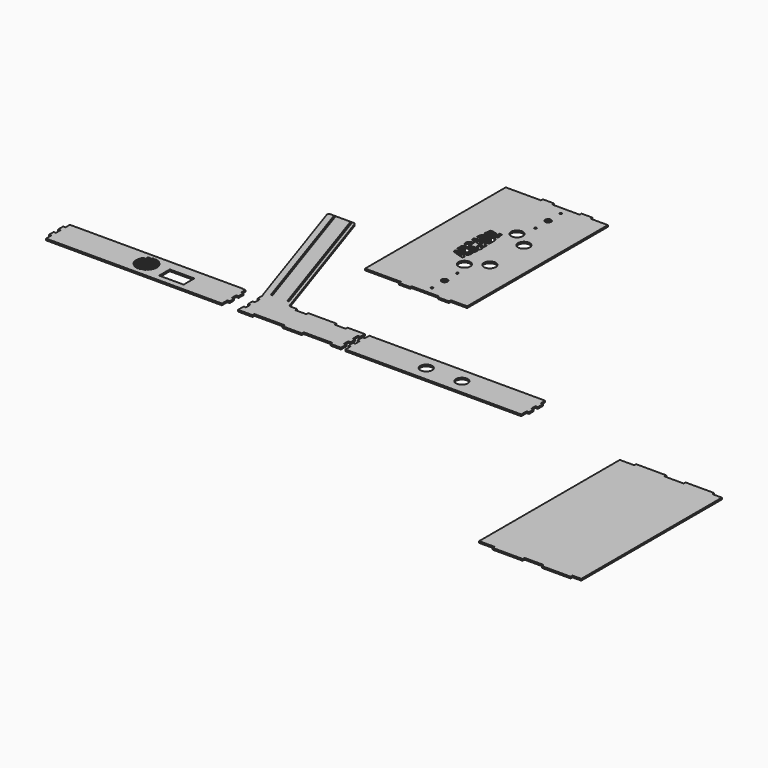
from build123d import *

# Parameters (mm, degrees)
F1_DEPTH = 4.45
F0_R     = 3
F0_R_2   = 8.087272744
F0_R_3   = 16.129
F0_W     = 66.7005181313
F0_H     = 36.3053381443


# Not quite as in the source:
# - ends of sketch curves that miss each other by under 0.0002 mm in the source are joined
# - a feature names something its author has since deleted; it is built from what else it names


with BuildPart() as f1:
    # F0 (on Top) → F1 (new body)
    with BuildSketch(Plane.XY):
        with BuildLine():
            Line((-13.1345508408, -164.6919741164), (-133.2231766972, 195.5739079059))
            ThreePointArc((-133.2231766972, 195.5739079059), (-135.0430417624, 198.0489800139), (-137.9665931933, 198.9927690934))
            Line((-137.9665931933, 198.9927690934), (-188.0199429035, 198.9927690934))
            Line((-188.0199429035, 198.9927690934), (-201.6566259516, 198.9927690934))
            ThreePointArc((-201.6566259516, 198.9927690934), (-205.7128368721, 196.9163205243), (-206.4000424478, 192.4116302809))
            Line((-206.4000424478, 192.4116302809), (-83.9924133672, -174.8112615001))
            Line((-83.9924133672, -174.8112615001), (-80.8544035681, -184.2252910137))
            Line((-80.8544035681, -184.2252910137), (-80.3456279762, -184.2252910137))
            Line((-80.3456279762, -184.2252910137), (-80.3456279762, -185.1425599537))
            Line((-80.3456279762, -185.1425599537), (-80.3456279762, -185.7516178083))
            Line((-80.3456279762, -185.7516178083), (-80.3456279762, -200.4338326941))
            Line((-80.3456279762, -200.4338326941), (-74.0156279762, -200.4338326941))
            Line((-74.0156279762, -200.4338326941), (-74.0156279762, -217.4338326941))
            Line((-74.0156279762, -217.4338326941), (-80.3456279762, -217.4338326941))
            Line((-80.3456279762, -217.4338326941), (-80.3456279762, -232.7338326941))
            Line((-80.3456279762, -232.7338326941), (-74.0156279762, -232.7338326941))
            Line((-74.0156279762, -232.7338326941), (-74.0156279762, -247.7338326941))
            Line((-74.0156279762, -247.7338326941), (-80.3456279762, -247.7338326941))
            Line((-80.3456279762, -247.7338326941), (-80.3456279762, -248.7336844206))
            Line((-80.3456279762, -248.7336844206), (-80.3456279762, -266.7746841908))
            Line((-80.3456279762, -266.7746841908), (-40.9429369935, -266.7746841908))
            Line((-40.9429369935, -266.7746841908), (-40.9429369935, -260.4446841907))
            Line((-40.9429369935, -260.4446841907), (41.0570630065, -260.4446841907))
            Line((41.0570630065, -260.4446841907), (41.0570630065, -266.7746841907))
            Line((41.0570630065, -266.7746841907), (93.3570630065, -266.7746841908))
            Line((93.3570630065, -266.7746841908), (93.3570630065, -260.4446841907))
            Line((93.3570630065, -260.4446841907), (171.3570630065, -260.4446841907))
            Line((171.3570630065, -260.4446841907), (171.3570630065, -266.3669029788))
            Line((171.3570630065, -266.3669029788), (199.4763922948, -266.3669029788))
            Line((199.4763922948, -266.3669029788), (199.4763922948, -248.4938822837))
            Line((199.4763922948, -248.4938822837), (193.1463922948, -248.4938822837))
            Line((193.1463922948, -248.4938822837), (193.1463922948, -233.4938822837))
            Line((193.1463922948, -233.4938822837), (199.4763922948, -233.4938822837))
            Line((199.4763922948, -233.4938822837), (199.4763922948, -218.1938822837))
            Line((199.4763922948, -218.1938822837), (193.1463922948, -218.1938822837))
            Line((193.1463922948, -218.1938822837), (193.1463922948, -201.1938822837))
            Line((193.1463922948, -201.1938822837), (199.8516707594, -201.1938822837))
            Line((199.8516707594, -201.1938822837), (199.8516707594, -200.6451304226))
            Line((199.8516707594, -200.6451304226), (199.8516707594, -185.7516178083))
            Line((199.8516707594, -185.7516178083), (152.5814315498, -185.7516178083))
            Line((152.5814315498, -185.7516178083), (152.5876286626, -192.0816178083))
            Line((152.5876286626, -192.0816178083), (122.5876286626, -192.0816178083))
            Line((122.5876286626, -192.0816178083), (122.5814315498, -185.7516178083))
            Line((122.5814315498, -185.7516178083), (47.2814315498, -185.7516178083))
            Line((47.2814315498, -185.7516178083), (45.8255372941, -185.7516178083))
            Line((45.8255372941, -185.7516178083), (45.8255372941, -192.0816178083))
            Line((45.8255372941, -192.0816178083), (15.8255372941, -192.0816178083))
            Line((15.8255372941, -192.0816178083), (15.8255372941, -185.7516178083))
            Line((15.8255372941, -185.7516178083), (-2.5108735826, -185.7516178083))
            ThreePointArc((-2.5108735826, -185.7516178083), (-5.4344250134, -184.8078287287), (-7.2542900787, -182.3327566208))
            Line((-7.2542900787, -182.3327566208), (-13.1345508408, -164.6919741164))
        make_face()
        Polygon((-68.8909804744, -169.5191176128), (-129.5292109794, 12.3955761507), (-190.322441274, 194.7752692889), (-185.872441274, 194.7752692889), (-125.1567108742, 12.6280758381), (-125.0792109794, 12.3955761507), (-64.4409804744, -169.5191176128), align=None, mode=Mode.SUBTRACT)
        Polygon((-145.372441274, 194.7752760296), (-140.922441274, 194.7752760296), (-19.4909804744, -169.5191108722), (-23.9409804744, -169.5191108722), (-84.6567108742, 12.6280825787), align=None, mode=Mode.SUBTRACT)
    extrude(amount=F1_DEPTH)


with BuildPart() as f1b:
    # F0 (on Top) → F1, piece 2 (new body)
    with BuildSketch(Plane.XY):
        Polygon((109.6645991251, 49.936733744), (109.6645991251, 43.606733744), (139.9645991251, 43.606733744), (139.9645991251, 48.056733744), (214.9645991251, 48.056733744), (214.9645991251, 43.606733744), (245.2645991251, 43.606733744), (245.2645991251, 49.936733744), (289.7008654758, 49.936733744), (289.7008654758, 528.386733744), (243.2266908545, 528.386733744), (243.2266908545, 534.716733744), (212.9266908545, 534.716733744), (212.9266908545, 528.386733744), (137.9266908545, 528.386733744), (137.9266908545, 534.716733744), (107.6266908545, 534.716733744), (107.6266908545, 528.386733744), (86.1305896078, 528.386733744), (11.8996296078, 528.386733744), (11.8996296078, 49.936733744), (86.1305896078, 49.936733744), align=None)
        with Locations((178.3758481905, 69.173247926)):
            Circle(F0_R, mode=Mode.SUBTRACT)
        with Locations((178.3758481905, 112.373247926)):
            Circle(F0_R_2, mode=Mode.SUBTRACT)
        with Locations((178.3758481905, 155.573247926)):
            Circle(F0_R, mode=Mode.SUBTRACT)
        with Locations((164.4027125835, 197.3344986652)):
            Circle(F0_R_3, mode=Mode.SUBTRACT)
        Polygon((144.38024237, 234.2502108202), (142.1130604967, 234.2502108202), (138.3344314918, 233.0626404271), (137.7946220263, 226.9088669107), (141.0334490165, 226.3150817141), (143.4625692591, 226.3150817141), (141.843155764, 218.1914640949), (140.1157833561, 218.9197583482), (134.9876381382, 220.3772260234), (123.0039752945, 224.2638251171), (109.6707962379, 228.5822598622), (108.9690484032, 235.0599175677), (128.5639636144, 238.406707196), (142.6528625115, 241.9694183752), (145.8329220252, 241.9694183752), align=None, mode=Mode.SUBTRACT)
        with Locations((208.4719767734, 228.5822598622)):
            Circle(F0_R_3, mode=Mode.SUBTRACT)
        with BuildLine():
            add(Edge.make_bspline(
                [(128.5639636168, 260.5926792261), (126.6851334747, 261.6323850443), (125.1709058254, 262.4309195257), (123.2035912523, 262.8997626838)],
                knots=[0, 0, 0, 0, 0.1162972911, 0.1162972911, 0.1162972911, 0.1162972911], degree=3))
            add(Edge.make_bspline(
                [(131.0810425796, 258.8106178703), (130.4885197933, 259.5182474814), (129.4826550141, 260.0842943704), (128.5639636168, 260.5926792261)],
                knots=[0.9431341245, 0.9431341245, 0.9431341245, 0.9431341245, 1, 1, 1, 1], degree=3))
            Line((131.0810425796, 258.8106178703), (147.2951849037, 264.5332548154))
            Line((147.2951849037, 264.5332548154), (146.6391187302, 255.3441180101))
            Line((146.6391187302, 255.3441180101), (145.0819902192, 255.0326926987))
            Line((145.0819902192, 255.0326926987), (132.7204562794, 250.509393456))
            Line((132.7204562794, 250.509393456), (145.9027750667, 250.509393456))
            Line((145.9027750667, 250.509393456), (145.6217922195, 242.5632035718))
            Line((145.6217922195, 242.5632035718), (107.8536775567, 243.898710594))
            add(Edge.make_bspline(
                [(107.457601274, 243.9127161291), (107.5681389055, 243.8955344904), (107.7007268333, 243.8910975861), (107.8536775567, 243.898710594)],
                knots=[0.6431910445, 0.6431910445, 0.6431910445, 0.6431910445, 0.6525586544, 0.6525586544, 0.6525586544, 0.6525586544], degree=3))
            add(Edge.make_bspline(
                [(123.2035912523, 262.8997626838), (120.8214160248, 263.467473904), (114.6447375539, 263.6384105597), (104.4496833821, 259.1667517285), (108.5099601756, 247.3009629552), (106.515459915, 244.0591597631), (107.457601274, 243.9127161291)],
                knots=[0.1162972911, 0.1162972911, 0.1162972911, 0.1162972911, 0.2571189623, 0.4018084692, 0.5633484367, 0.6431910445, 0.6431910445, 0.6431910445, 0.6431910445], degree=3))
        make_face(mode=Mode.SUBTRACT)
        with BuildLine():
            add(Edge.make_bspline(
                [(118.4096939812, 278.2062657301), (118.008613675, 277.7544534713), (116.5254907196, 278.3846987718), (114.6860986223, 277.3704216428), (114.3121353636, 275.4818719009), (115.8822495107, 273.5639671058), (122.1543701521, 271.8085591307), (128.3372312156, 271.631565814), (134.6144229239, 272.2452065368), (138.281513843, 274.0041420395), (138.8901224926, 277.3280303811), (135.816879855, 277.8372704412), (132.3043819598, 278.6943910776), (132.8801296382, 279.7199041248), (133.0335295094, 286.4615207561), (131.517785638, 288.8097379759), (143.3081485383, 285.6706131454), (143.2876661042, 285.1920333687), (149.7203259126, 281.8270369122), (148.695702836, 273.0090093242), (145.8257996198, 267.8254041605), (137.5916580466, 263.7489152162), (126.7832057192, 262.9795878345), (114.9700731672, 264.1210882589), (108.486783454, 268.147637912), (104.5049371001, 272.096645925), (104.3359645468, 276.9661032929), (105.5397960824, 282.3849948376), (111.6880120097, 286.3382367425), (116.9904636561, 287.4430295691), (118.7674772932, 287.8835911533), (118.4200692992, 285.1487585296), (119.1960011795, 279.0920315629), (118.4096939812, 278.2062657301)],
                knots=[0, 0, 0, 0, 0.020494547, 0.0414693591, 0.0607350939, 0.0828404788, 0.1209521426, 0.159932456, 0.1980232824, 0.2276772762, 0.2510011815, 0.2764947931, 0.3037065377, 0.3173900946, 0.3574312462, 0.3741991924, 0.4232910827, 0.4368372532, 0.4735096835, 0.516799885, 0.5533151147, 0.5976483724, 0.648419728, 0.7005614172, 0.7421530316, 0.776720808, 0.8090959926, 0.8438514827, 0.8845213381, 0.9201032118, 0.9362852602, 0.9598209895, 1, 1, 1, 1], degree=3))
        make_face(mode=Mode.SUBTRACT)
        Polygon((146.2362490544, 313.2235731122), (146.9237737307, 313.160742366), (146.9237737307, 304.04164336), (144.6443654547, 304.04164336), (140.3559751758, 303.0352617738), (140.3559751758, 296.2421939832), (145.2770911107, 294.9842183974), (147.5267268667, 294.9842183974), (147.5016705642, 285.6739075454), (105.6019298682, 295.4861174461), (105.6019298682, 302.4049817708), align=None, mode=Mode.SUBTRACT)
        with BuildLine():
            ThreePointArc((107.1513079057, 320.8409628955), (125.426885077, 335.327875154), (146.2362490544, 324.7999257532))
            Line((146.2362490544, 324.7999257532), (146.9237737307, 313.6994063047))
            Line((146.9237737307, 313.6994063047), (106.4939506302, 312.5978863922))
            Line((106.4939506302, 312.5978863922), (107.1513079057, 320.8409628955))
        make_face(mode=Mode.SUBTRACT)
        Polygon((130.0334616295, 350.7802296276), (131.2729376142, 342.1865778554), (135.6725178609, 342.8211362717), (134.1524355063, 353.3603145865), (141.6923932681, 353.3603145865), (143.9817920473, 337.2012575192), (108.2818875652, 334.854008616), (111.446634675, 352.6165901807), (119.4676615248, 353.1822159079), (117.2535054335, 341.9162227896), (122.8425063143, 341.9162227896), (122.8425063143, 350.7802296276), align=None, mode=Mode.SUBTRACT)
        with Locations((208.4719767734, 344.6277944729)):
            Circle(F0_R_3, mode=Mode.SUBTRACT)
        with Locations((164.4027125835, 375.8755556698)):
            Circle(F0_R_3, mode=Mode.SUBTRACT)
        with Locations((178.3758481905, 421.2868064091)):
            Circle(F0_R, mode=Mode.SUBTRACT)
        with Locations((178.3758481905, 464.4868064091)):
            Circle(F0_R_2, mode=Mode.SUBTRACT)
        with Locations((178.3758481905, 507.6868064091)):
            Circle(F0_R, mode=Mode.SUBTRACT)
        with BuildLine():
            Line((128.5639636168, 260.5926792261), (130.7771585832, 258.7033647236))
            Line((130.7771585832, 258.7033647236), (131.0810425796, 258.8106178703))
            add(Edge.make_bspline(
                [(131.0810425796, 258.8106178703), (130.4885197933, 259.5182474814), (129.4826550141, 260.0842943704), (128.5639636168, 260.5926792261)],
                knots=[0.9431341245, 0.9431341245, 0.9431341245, 0.9431341245, 1, 1, 1, 1], degree=3))
        make_face()
    extrude(amount=F1_DEPTH)


with BuildPart() as f1c:
    # F0 (on Top) → F1, piece 3 (new body)
    with BuildSketch(Plane.XY):
        Polygon((121.6972161211, 253.4000544932), (120.1217256436, 254.4976013836), (118.3763080916, 254.3745182559), (117.2535054335, 254.0755802312), (116.3434170136, 253.4000544932), (115.9999452481, 250.6342387882), (121.6972161211, 250.4327792945), align=None)
    extrude(amount=F1_DEPTH)


with BuildPart() as f1d:
    # F0 (on Top) → F1, piece 4 (new body)
    with BuildSketch(Plane.XY):
        Polygon((125.6387986193, 230.2756949452), (129.8662058959, 228.9461760905), (129.8662058959, 231.1009175268), align=None)
    extrude(amount=F1_DEPTH)


with BuildPart() as f1e:
    # F0 (on Top) → F1, piece 5 (new body)
    with BuildSketch(Plane.XY):
        Polygon((130.8137707362, 300.8135954973), (125.054859365, 299.5041205671), (130.8137707362, 298.1946465683), align=None)
    extrude(amount=F1_DEPTH)


with BuildPart() as f1f:
    # F0 (on Top) → F1, piece 6 (new body)
    with BuildSketch(Plane.XY):
        with BuildLine():
            Line((117.2535054335, 321.2757527021), (135.9537251243, 321.2757527021))
            Line((135.9537251243, 321.2757527021), (135.6725178609, 323.917501339))
            ThreePointArc((135.6725178609, 323.917501339), (126.3572301292, 327.5379858027), (117.2535054335, 323.4143114772))
            Line((117.2535054335, 323.4143114772), (117.2535054335, 321.2757527021))
        make_face()
    extrude(amount=F1_DEPTH)


with BuildPart() as f1g:
    # F0 (on Top) → F1, piece 7 (new body)
    with BuildSketch(Plane.XY):
        Polygon((690.2977205402, -185.7516178083), (211.8477205402, -185.7516178083), (211.8477205402, -200.6451304226), (211.8477205402, -200.8938822837), (205.5177205402, -200.8938822837), (205.5177205402, -218.1938822837), (211.8477205402, -218.1938822837), (211.8477205402, -226.2631509995), (211.8477205402, -230.1938822837), (211.8477205402, -232.7680322837), (211.8477205402, -233.1938822837), (205.5161595345, -233.1938822837), (205.5161595345, -248.4938822837), (211.8477205402, -248.4938822837), (211.8477205402, -266.7746841908), (690.2977205402, -266.7746841908), (690.2977205402, -248.4956532717), (696.6277205402, -248.4956532717), (696.6277205402, -233.1956532717), (690.2977205402, -233.1956532717), (690.2977205402, -218.1956532717), (696.6277205402, -218.1956532717), (696.6277205402, -200.8956532717), (690.2977205402, -200.8956532717), align=None)
        with Locations((399.4364652282, -226.2631509995)):
            Circle(F0_R_3, mode=Mode.SUBTRACT)
        with Locations((496.3774148464, -226.2631509995)):
            Circle(F0_R_3, mode=Mode.SUBTRACT)
    extrude(amount=F1_DEPTH)


with BuildPart() as f1h:
    # F0 (on Top) → F1, piece 8 (new body)
    with BuildSketch(Plane.XY):
        Polygon((-133.2186609507, -184.645057578), (-603.5792125037, -184.645057578), (-603.5792125037, -199.7890930414), (-609.9092125037, -199.7890930414), (-609.9092125037, -217.0890930414), (-603.5792125037, -217.0890930414), (-603.5792125037, -232.0890930414), (-609.9092125037, -232.0890930414), (-609.9092125037, -247.3890930414), (-603.5792125037, -247.3890930414), (-603.5792125037, -265.6681239605), (-125.0792125037, -265.6681239605), (-125.0792125037, -247.3890930414), (-118.7492125037, -247.3890930414), (-118.7492125037, -232.0890930414), (-125.0792125037, -232.0890930414), (-125.0792125037, -229.0384530414), (-125.0792125037, -217.0890930414), (-118.7492125037, -217.0890930414), (-118.7492125037, -199.7890930414), (-125.0792125037, -199.7890930414), (-125.0792125037, -185.7516178083), (-133.2186609507, -185.7516178083), align=None)
        with BuildLine():
            Line((-383.3327464205, -202.6777080565), (-383.3327464205, -243.4498380263))
            ThreePointArc((-383.3327464205, -243.4498380263), (-392.1990159996, -223.0637730414), (-383.3327464205, -202.6777080565))
        make_face(mode=Mode.SUBTRACT)
        with BuildLine():
            Line((-373.5705486876, -196.7707387465), (-373.5705486876, -249.3568073363))
            ThreePointArc((-373.5705486876, -249.3568073363), (-377.1578306316, -247.805488904), (-380.4928235156, -245.7675970795))
            Line((-380.4928235156, -245.7675970795), (-380.4928235156, -200.3599490033))
            ThreePointArc((-380.4928235156, -200.3599490033), (-377.4663403703, -197.7270546447), (-373.5705486876, -196.7707387465))
        make_face(mode=Mode.SUBTRACT)
        with BuildLine():
            Line((-365.7607905013, -195.2307615024), (-365.7607905013, -250.8967845805))
            ThreePointArc((-365.7607905013, -250.8967845805), (-368.261689351, -250.6547420846), (-370.7306257826, -250.1884454805))
            Line((-370.7306257826, -250.1884454805), (-370.7306257826, -195.9391006023))
            ThreePointArc((-370.7306257826, -195.9391006023), (-368.261689351, -195.4728039983), (-365.7607905013, -195.2307615024))
        make_face(mode=Mode.SUBTRACT)
        with BuildLine():
            ThreePointArc((-362.8976345062, -195.2307615024), (-360.3967356565, -195.4728039983), (-357.9277992249, -195.9391006023))
            Line((-357.9277992249, -195.9391006023), (-357.9277992249, -250.1884454805))
            ThreePointArc((-357.9277992249, -250.1884454805), (-360.3967356565, -250.6547420846), (-362.8976345062, -250.8967845805))
            Line((-362.8976345062, -250.8967845805), (-362.8976345062, -195.2307615024))
        make_face(mode=Mode.SUBTRACT)
        with BuildLine():
            ThreePointArc((-348.1656014919, -245.7675970795), (-351.5005943759, -247.805488904), (-355.0878763199, -249.3568073363))
            Line((-355.0878763199, -249.3568073363), (-355.0878763199, -196.7707387465))
            ThreePointArc((-355.0878763199, -196.7707387465), (-351.5005943759, -198.3220571788), (-348.1656014919, -200.3599490033))
            Line((-348.1656014919, -200.3599490033), (-348.1656014919, -245.7675970795))
        make_face(mode=Mode.SUBTRACT)
        with BuildLine():
            Line((-345.325678587, -243.4498380263), (-345.325678587, -202.6777080565))
            ThreePointArc((-345.325678587, -202.6777080565), (-336.4594090079, -223.0637730414), (-345.325678587, -243.4498380263))
        make_face(mode=Mode.SUBTRACT)
        with Locations((-276.2150764465, -230.4605394602)):
            Rectangle(F0_W, F0_H, mode=Mode.SUBTRACT)
    extrude(amount=F1_DEPTH)


with BuildPart() as f1i:
    # F0 (on Top) → F1, piece 9 (new body)
    with BuildSketch(Plane.XY):
        Polygon((1023.8570030112, -299.4968297958), (984.6543073654, -299.4968297958), (984.6543073654, -773.4968297958), (984.6543073654, -777.9468297958), (1026.0729903258, -777.9468297958), (1026.0729903258, -784.2768297958), (1108.3729903258, -784.2768297958), (1108.3729903258, -777.9468297958), (1160.3729903258, -777.9468297958), (1160.3729903258, -784.2768297958), (1238.6729903258, -784.2768297958), (1238.6729903258, -777.9468297958), (1262.4696718737, -777.9468297958), (1262.4696718737, -299.4968297958), (1240.658860787, -299.4968297958), (1236.4570030112, -299.4968297958), (1236.4570030112, -293.1668297958), (1158.1570030112, -293.1668297958), (1158.1570030112, -299.4968297958), (1106.1570030112, -299.4968297958), (1106.1570030112, -293.1668297958), (1023.8570030112, -293.1668297958), align=None)
    extrude(amount=F1_DEPTH)


solid = Compound([f1.part, f1b.part, f1c.part, f1d.part, f1e.part, f1f.part, f1g.part, f1h.part, f1i.part])
